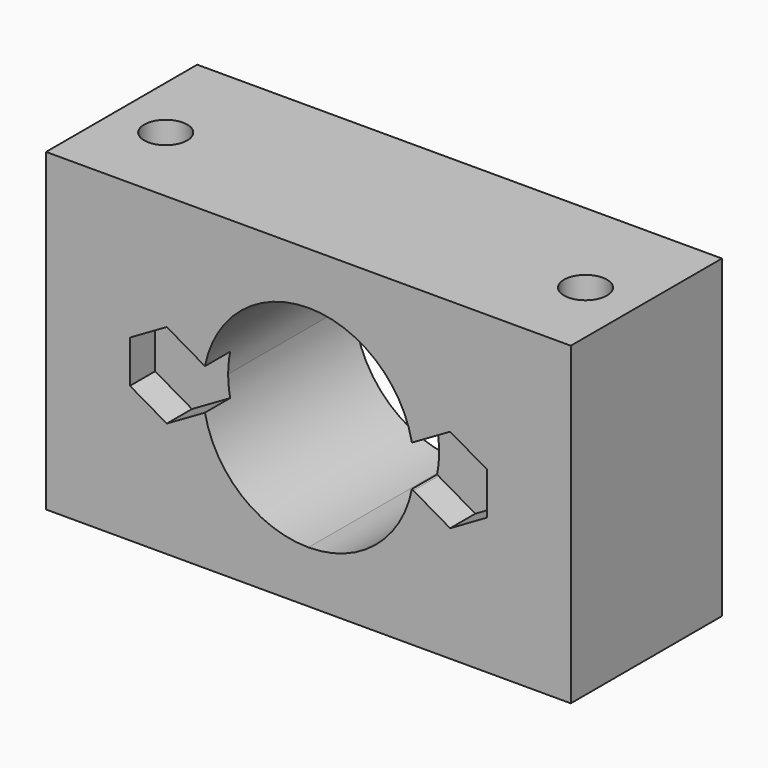
from build123d import *

# Parameters (mm, degrees)
F0_R      = 2.05
F1_DEPTH  = 18
F3_DEPTH  = 30
F4_R      = 3.5
F5_DEPTH  = 5
F7_DEPTH  = 3
F8_R      = 2.05
F9_R      = 2.05
F10_DEPTH = 0.4


with BuildPart() as f1:
    # F0 (on Front) → F1 (new body)
    with BuildSketch(Plane.XZ):
        with BuildLine():
            ThreePointArc((0, 10.05), (7.1064231509, 7.1064231509), (10.05, 0))
            ThreePointArc((10.05, 0), (7.1064231509, -7.1064231509), (0, -10.05))
            Line((0, -10.05), (0, -15))
            Line((0, -15), (25, -15))
            Line((25, -15), (25, 0))
            Line((25, 0), (25, 15))
            Line((25, 15), (0, 15))
            Line((0, 15), (0, 10.05))
        make_face()
        with BuildLine():
            ThreePointArc((15.55, 0), (13.5, -2.05), (11.45, 0))
            ThreePointArc((11.45, 0), (13.5, 2.05), (15.55, 0))
        make_face(mode=Mode.SUBTRACT)
        with BuildLine():
            ThreePointArc((-10.05, 0), (-7.1064231509, 7.1064231509), (0, 10.05))
            Line((0, 10.05), (0, 15))
            Line((0, 15), (-25, 15))
            Line((-25, 15), (-25, 0))
            Line((-25, 0), (-25, -15))
            Line((-25, -15), (0, -15))
            Line((0, -15), (0, -10.05))
            ThreePointArc((0, -10.05), (-7.1064231509, -7.1064231509), (-10.05, 0))
        make_face()
        with Locations((-13.5, 0)):
            Circle(F0_R, mode=Mode.SUBTRACT)
    extrude(amount=F1_DEPTH)

    # F2 (on face) → F3 (cut)
    with BuildSketch(Plane(origin=(0, 0, -15), x_dir=(1, 0, 0), z_dir=(0, 0, -1))):
        with BuildLine():
            ThreePointArc((17.95, 10), (20, 7.95), (22.05, 10))
            Line((22.05, 10), (17.95, 10))
        make_face()
        with BuildLine():
            Line((17.95, 10), (22.05, 10))
            ThreePointArc((22.05, 10), (20, 12.05), (17.95, 10))
        make_face()
        with BuildLine():
            ThreePointArc((-17.95, 10), (-20, 12.05), (-22.05, 10))
            Line((-22.05, 10), (-17.95, 10))
        make_face()
        with BuildLine():
            Line((-17.95, 10), (-22.05, 10))
            ThreePointArc((-22.05, 10), (-20, 7.95), (-17.95, 10))
        make_face()
    extrude(amount=-F3_DEPTH, mode=Mode.SUBTRACT)

    # F4 (on face) → F5 (cut)
    with BuildSketch(Plane(origin=(0, 0, -15), x_dir=(1, 0, 0), z_dir=(0, 0, -1))):
        with Locations((20, 10)):
            Circle(F4_R)
        with Locations((-20, 10)):
            Circle(F4_R)
    extrude(amount=-F5_DEPTH, mode=Mode.SUBTRACT)

    # F6 (on face) → F7 (cut)
    with BuildSketch(Plane.XZ.offset(18)):
        Polygon((-13.5, 4.05), (-13.5, 0), (-13.5, -4.05), (-9.9925971147, -2.025), (-7.9662247081, -0.8550733456), (-7.7903810671, 0.7535499721), (-9.9925971147, 2.025), align=None)
        Polygon((-13.5, -4.05), (-13.5, 0), (-13.5, 4.05), (-17.0074028853, 2.025), (-17.0074028853, -2.025), align=None)
        Polygon((13.5, -4.05), (13.5, 0), (13.5, 4.05), (9.9925971147, 2.025), (9.9925971147, -2.025), align=None)
        Polygon((13.5, 4.05), (13.5, 0), (13.5, -4.05), (17.0074028853, -2.025), (17.0074028853, 2.025), align=None)
        Polygon((9.9925971147, -2.025), (9.9925971147, 2.025), (7.4926645733, 0.5816632743), (7.2557264377, -0.4448669779), align=None)
    extrude(amount=-F7_DEPTH, mode=Mode.SUBTRACT)

    # F8 (on face) + F9 (on face) → F10 (join)
    with BuildSketch(Plane.XZ.offset(15)):
        with Locations((13.5, 0)):
            Circle(F8_R)
    with BuildSketch(Plane.XZ.offset(15)):
        with Locations((-13.5, 0)):
            Circle(F9_R)
    extrude(amount=-F10_DEPTH)


solid = f1.part
